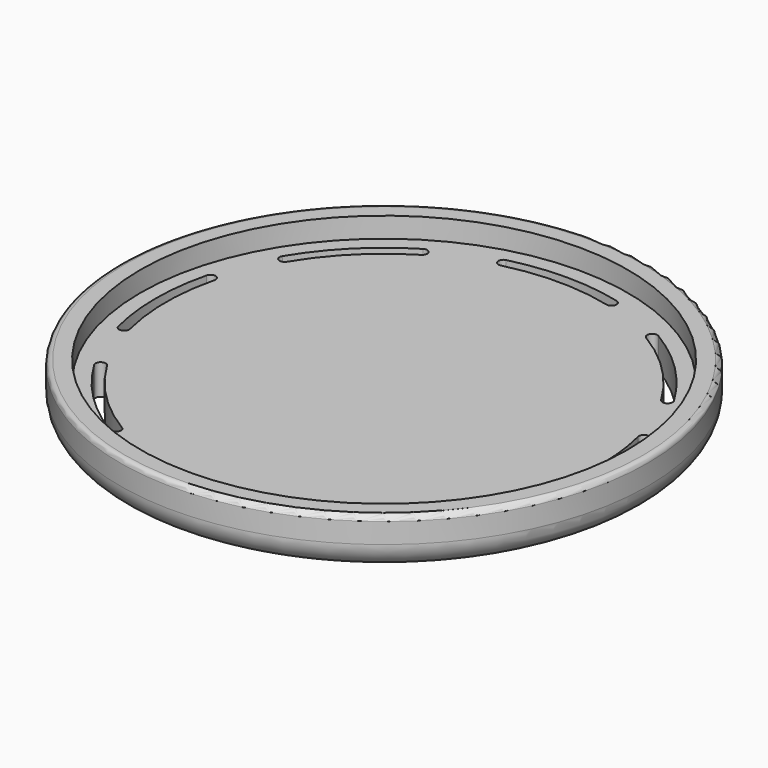
from build123d import *

# Parameters (mm, degrees)
F1_START = 3
F0_R     = 26
F0_R_2   = 24
F1_DEPTH = 2
F0_R_3   = 20.5
F0_R_4   = 16.5
F2_DEPTH = 3
F3_R     = 2.5
F4_R     = 0.5
F5_DEPTH = 0.3


with BuildPart() as f1:
    # F0 (on Top) → F1 (new body)
    with BuildSketch(Plane.XY.offset(F1_START)):
        Circle(F0_R)
        Circle(F0_R_2, mode=Mode.SUBTRACT)
    extrude(amount=F1_DEPTH)

    # F0 (on Top) → F2 (join)
    with BuildSketch(Plane.XY):
        Circle(F0_R)
        Circle(F0_R_2, mode=Mode.SUBTRACT)
        Circle(F0_R_2)
        with BuildLine():
            ThreePointArc((21.8316538648, 5.4432425563), (22.3322884179, 2.7420601782), (22.5, 0))
            ThreePointArc((22.5, 0), (22.3322884062, -2.7420602736), (21.8316538183, -5.4432427429))
            ThreePointArc((21.8316538183, -5.4432427429), (20.7872894705, -8.6103772548), (19.286264285, -11.5883566536))
            ThreePointArc((19.286264285, -11.5883566536), (15.9099025767, -15.9099025767), (11.5883566536, -19.286264285))
            ThreePointArc((11.5883566536, -19.286264285), (8.6103771829, -20.7872895003), (5.4432425919, -21.8316538559))
            ThreePointArc((5.4432425919, -21.8316538559), (7e-09, -22.5), (-5.4432425783, -21.8316538593))
            ThreePointArc((-5.4432425783, -21.8316538593), (-8.6103772201, -20.7872894849), (-11.5883567347, -19.2862642362))
            ThreePointArc((-11.5883567347, -19.2862642362), (-15.9099026102, -15.9099025432), (-19.286264285, -11.5883566536))
            ThreePointArc((-19.286264285, -11.5883566536), (-20.7872895003, -8.6103771829), (-21.8316538559, -5.4432425919))
            ThreePointArc((-21.8316538559, -5.4432425919), (-22.5, 6.65e-08), (-21.8316538238, 5.4432427209))
            ThreePointArc((-21.8316538238, 5.4432427209), (-20.7872894493, 8.610377306), (-19.2862642162, 11.5883567681))
            ThreePointArc((-19.2862642162, 11.5883567681), (-15.9099025183, 15.9099026351), (-11.5883566265, 19.2862643012))
            ThreePointArc((-11.5883566265, 19.2862643012), (-8.6103772402, 20.7872894765), (-5.4432427429, 21.8316538183))
            ThreePointArc((-5.4432427429, 21.8316538183), (-7.78e-08, 22.5), (5.4432425919, 21.8316538559))
            ThreePointArc((5.4432425919, 21.8316538559), (8.6103771829, 20.7872895003), (11.5883566536, 19.286264285))
            ThreePointArc((11.5883566536, 19.286264285), (15.9099025587, 15.9099025947), (19.2862642587, 11.5883566973))
            ThreePointArc((19.2862642587, 11.5883566973), (20.7872894975, 8.6103771895), (21.8316538648, 5.4432425563))
        make_face(mode=Mode.SUBTRACT)
        with BuildLine():
            ThreePointArc((21.5, 0), (21.3397422613, 2.6201908748), (20.861358119, 5.201320739))
            ThreePointArc((20.861358119, 5.201320739), (19.8634099525, 8.2276937874), (18.4290969658, 11.0733186094))
            ThreePointArc((18.4290969658, 11.0733186094), (15.2027957959, 15.2027957951), (11.0733186103, 18.4290969652))
            ThreePointArc((11.0733186103, 18.4290969652), (8.2276938087, 19.8634099437), (5.2013207828, 20.8613581081))
            ThreePointArc((5.2013207828, 20.8613581081), (1.96e-08, 21.5), (-5.2013207448, 20.8613581176))
            ThreePointArc((-5.2013207448, 20.8613581176), (-8.2276937956, 19.8634099491), (-11.0733186195, 18.4290969597))
            ThreePointArc((-11.0733186195, 18.4290969597), (-15.2027957888, 15.2027958023), (-18.4290969499, 11.0733186359))
            ThreePointArc((-18.4290969499, 11.0733186359), (-19.8634099566, 8.2276937776), (-20.8613581316, 5.2013206884))
            ThreePointArc((-20.8613581316, 5.2013206884), (-21.5, -2.91e-08), (-20.8613581176, -5.2013207448))
            ThreePointArc((-20.8613581176, -5.2013207448), (-19.8634099536, -8.2276937847), (-18.4290969719, -11.0733185993))
            ThreePointArc((-18.4290969719, -11.0733185993), (-15.2027958064, -15.2027957846), (-11.0733186258, -18.429096956))
            ThreePointArc((-11.0733186258, -18.429096956), (-8.227693799, -19.8634099477), (-5.2013207448, -20.8613581176))
            ThreePointArc((-5.2013207448, -20.8613581176), (0, -21.5), (5.2013207448, -20.8613581176))
            ThreePointArc((5.2013207448, -20.8613581176), (8.227693799, -19.8634099477), (11.0733186258, -18.429096956))
            ThreePointArc((11.0733186258, -18.429096956), (15.2027957955, -15.2027957955), (18.429096956, -11.0733186258))
            ThreePointArc((18.429096956, -11.0733186258), (19.8634099351, -8.2276938293), (20.8613581017, -5.2013208084))
            ThreePointArc((20.8613581017, -5.2013208084), (21.339742257, -2.6201909103), (21.5, 0))
        make_face()
        Circle(F0_R_3, mode=Mode.SUBTRACT)
        Circle(F0_R_3)
        Circle(F0_R_4, mode=Mode.SUBTRACT)
        Circle(F0_R_4)
        with BuildLine():
            ThreePointArc((-18.4290969499, 11.0733186359), (-19.1151996816, 10.9022540149), (-19.2862642162, 11.5883567681))
            ThreePointArc((-19.2862642162, 11.5883567681), (-20.7872894493, 8.610377306), (-21.8316538238, 5.4432427209))
            ThreePointArc((-21.8316538238, 5.4432427209), (-21.2855712706, 5.8185547746), (-20.8465059781, 5.3222817032))
            ThreePointArc((-20.8465059781, 5.3222817032), (-20.8502329065, 5.2613469972), (-20.8613581316, 5.2013206884))
            ThreePointArc((-20.8613581316, 5.2013206884), (-19.8634099566, 8.2276937776), (-18.4290969499, 11.0733186359))
        make_face()
        with BuildLine():
            ThreePointArc((-5.2013207448, 20.8613581176), (-5.8074295536, 21.225544979), (-5.4432427429, 21.8316538183))
            ThreePointArc((-5.4432427429, 21.8316538183), (-8.6103772402, 20.7872894765), (-11.5883566265, 19.2862643012))
            ThreePointArc((-11.5883566265, 19.2862643012), (-11.084625838, 19.2928584465), (-10.830837648, 18.8576806154))
            ThreePointArc((-10.830837648, 18.8576806154), (-10.8956598026, 18.6114688309), (-11.0733186195, 18.4290969597))
            ThreePointArc((-11.0733186195, 18.4290969597), (-8.2276937956, 19.8634099491), (-5.2013207448, 20.8613581176))
        make_face()
        with BuildLine():
            ThreePointArc((11.0733186103, 18.4290969652), (10.9022539882, 19.1151996371), (11.5883566536, 19.286264285))
            ThreePointArc((11.5883566536, 19.286264285), (8.6103771829, 20.7872895003), (5.4432425919, 21.8316538559))
            ThreePointArc((5.4432425919, 21.8316538559), (5.7162870612, 21.6543367397), (5.8222817032, 21.3465059781))
            ThreePointArc((5.8222817032, 21.3465059781), (5.630112452, 20.95250061), (5.2013207828, 20.8613581081))
            ThreePointArc((5.2013207828, 20.8613581081), (8.2276938087, 19.8634099437), (11.0733186103, 18.4290969652))
        make_face()
        with BuildLine():
            ThreePointArc((20.861358119, 5.201320739), (21.2255450694, 5.8074295761), (21.8316538648, 5.4432425563))
            ThreePointArc((21.8316538648, 5.4432425563), (20.7872894975, 8.6103771895), (19.2862642587, 11.5883566973))
            ThreePointArc((19.2862642587, 11.5883566973), (19.3394958402, 11.4644568427), (19.3576806154, 11.330837648))
            ThreePointArc((19.3576806154, 11.330837648), (18.9912998041, 10.8490224216), (18.4290969658, 11.0733186094))
            ThreePointArc((18.4290969658, 11.0733186094), (19.8634099525, 8.2276937874), (20.861358119, 5.201320739))
        make_face()
        with BuildLine():
            ThreePointArc((19.286264285, -11.5883566536), (20.7872894705, -8.6103772548), (21.8316538183, -5.4432427429))
            ThreePointArc((21.8316538183, -5.4432427429), (21.2255450109, -5.8074295615), (20.8613581017, -5.2013208084))
            ThreePointArc((20.8613581017, -5.2013208084), (19.8634099351, -8.2276938293), (18.429096956, -11.0733186258))
            ThreePointArc((18.429096956, -11.0733186258), (18.9912997949, -10.849022419), (19.3576806154, -11.330837648))
            ThreePointArc((19.3576806154, -11.330837648), (19.339495847, -11.4644568181), (19.286264285, -11.5883566536))
        make_face()
        with BuildLine():
            ThreePointArc((5.4432425919, -21.8316538559), (8.6103771829, -20.7872895003), (11.5883566536, -19.286264285))
            ThreePointArc((11.5883566536, -19.286264285), (10.9022539835, -19.1151996293), (11.0733186258, -18.429096956))
            ThreePointArc((11.0733186258, -18.429096956), (8.227693799, -19.8634099477), (5.2013207448, -20.8613581176))
            ThreePointArc((5.2013207448, -20.8613581176), (5.6301124365, -20.9525005979), (5.8222817032, -21.3465059781))
            ThreePointArc((5.8222817032, -21.3465059781), (5.7162870612, -21.6543367397), (5.4432425919, -21.8316538559))
        make_face()
        with BuildLine():
            ThreePointArc((-11.5883567347, -19.2862642362), (-8.6103772201, -20.7872894849), (-5.4432425783, -21.8316538593))
            ThreePointArc((-5.4432425783, -21.8316538593), (-5.8074295741, -21.2255450613), (-5.2013207448, -20.8613581176))
            ThreePointArc((-5.2013207448, -20.8613581176), (-8.227693799, -19.8634099477), (-11.0733186258, -18.429096956))
            ThreePointArc((-11.0733186258, -18.429096956), (-10.8956598044, -18.6114688277), (-10.830837648, -18.8576806154))
            ThreePointArc((-10.830837648, -18.8576806154), (-11.0846258929, -19.2928584775), (-11.5883567347, -19.2862642362))
        make_face()
        with BuildLine():
            ThreePointArc((-21.8316538559, -5.4432425919), (-20.7872895003, -8.6103771829), (-19.286264285, -11.5883566536))
            ThreePointArc((-19.286264285, -11.5883566536), (-19.1151996426, -10.9022539915), (-18.4290969719, -11.0733185993))
            ThreePointArc((-18.4290969719, -11.0733185993), (-19.8634099536, -8.2276937847), (-20.8613581176, -5.2013207448))
            ThreePointArc((-20.8613581176, -5.2013207448), (-20.8502329029, -5.2613470261), (-20.8465059781, -5.3222817032))
            ThreePointArc((-20.8465059781, -5.3222817032), (-21.2855713366, -5.8185547827), (-21.8316538559, -5.4432425919))
        make_face()
    extrude(amount=F2_DEPTH)

    # F3
    f3_edges = [f1.edges().sort_by_distance(p)[0] for p in [
        (-26, 0, 0),
    ]]
    fillet(f3_edges, radius=F3_R)

    # F4
    f4_edges = [f1.edges().sort_by_distance(p)[0] for p in [
        (-26, 0, 5),
    ]]
    fillet(f4_edges, radius=F4_R)


with BuildPart() as f5:
    # F0 (on Top) → F5 (new body)
    with BuildSketch(Plane.XY):
        Circle(F0_R_3)
        Circle(F0_R_4, mode=Mode.SUBTRACT)
    extrude(amount=-F5_DEPTH)


solid = Compound([f1.part, f5.part])
